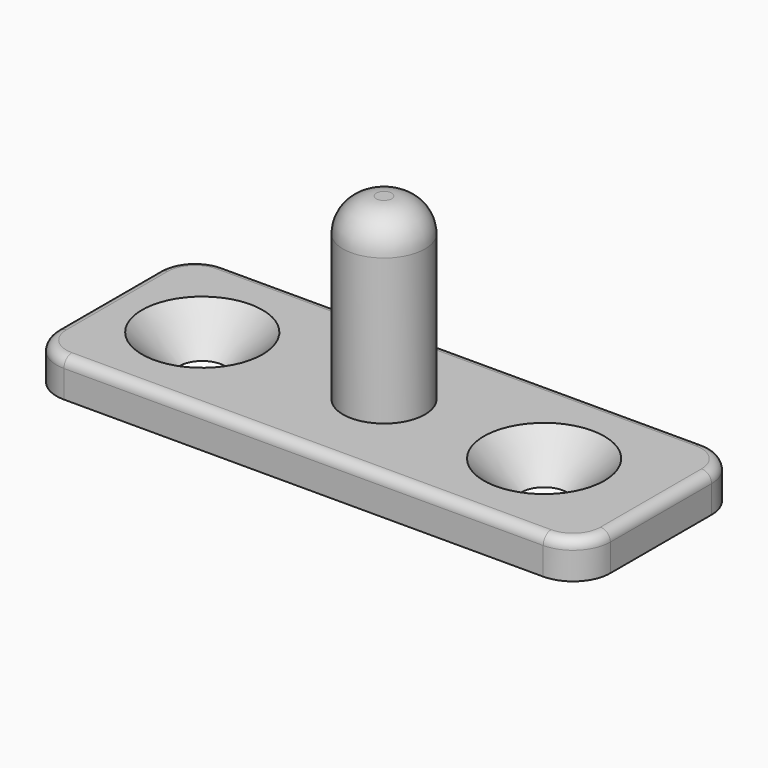
from build123d import *

# Parameters (mm, degrees)
F0_R     = 2.794
F1_DEPTH = 14.732
F0_W     = 37.719
F0_H     = 13.6906
F0_R_2   = 1.5621
F2_DEPTH = 2.54
F3_SIZE  = 2.53999
F4_R     = 2.54
F5_R     = 2.2688779059
F6_R     = 0.6745312693


# Not quite as in the source:
# - a fillet or chamfer is up to 0.001 mm smaller than in the source, because OpenCascade refuses the exact size


with BuildPart() as f1:
    # F0 (on Top) → F1 (new body)
    with BuildSketch(Plane.XY):
        Circle(F0_R)
    extrude(amount=F1_DEPTH)

    # F0 (on Top) → F2 (join)
    with BuildSketch(Plane.XY):
        Rectangle(F0_W, F0_H)
        with Locations((-12.3765456688, 0)):
            Circle(F0_R_2, mode=Mode.SUBTRACT)
        Circle(F0_R, mode=Mode.SUBTRACT)
        with Locations((10.9031473519, 0)):
            Circle(F0_R_2, mode=Mode.SUBTRACT)
    extrude(amount=F2_DEPTH)

    # F3 (size 2.54 in the source; OpenCascade refuses exactly that, so slightly less here)
    f3_edges = [f1.edges().sort_by_distance(p)[0] for p in [
        (-13.938646, 0, 2.54),
        (9.341047, 0, 2.54),
    ]]
    chamfer(f3_edges, length=F3_SIZE)

    # F4
    f4_edges = [f1.edges().sort_by_distance(p)[0] for p in [
        (18.8595, -6.8453, 1.27),
        (18.8595, 6.8453, 1.27),
        (-18.8595, -6.8453, 1.27),
        (-18.8595, 6.8453, 1.27),
    ]]
    fillet(f4_edges, radius=F4_R)

    # F5
    f5_edges = [f1.edges().sort_by_distance(p)[0] for p in [
        (-2.794, 0, 14.732),
    ]]
    fillet(f5_edges, radius=F5_R)

    # F6
    f6_edges = [f1.edges().sort_by_distance(p)[0] for p in [
        (0, -6.8453, 2.54),
        (18.115551, -6.101351, 2.54),
        (18.8595, 0, 2.54),
        (0, 6.8453, 2.54),
        (18.115551, 6.101351, 2.54),
        (-18.115551, 6.101351, 2.54),
        (-18.8595, 0, 2.54),
        (-18.115551, -6.101351, 2.54),
    ]]
    fillet(f6_edges, radius=F6_R)


solid = f1.part
